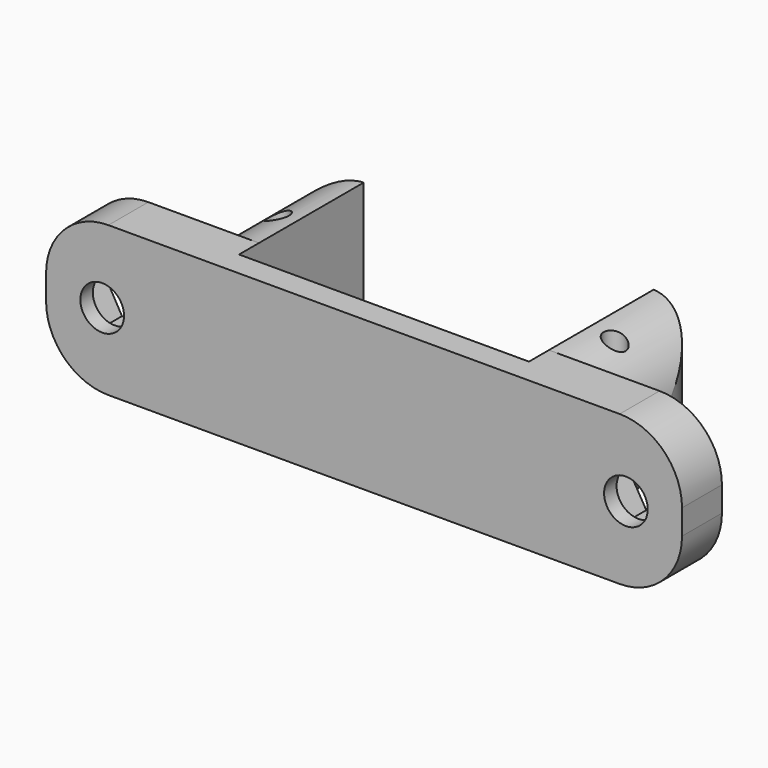
from build123d import *

# Parameters (mm, degrees)
F0_R        = 0.875
F1_DEPTH    = 12
F2_R        = 1.75
F3_DEPTH    = 25
F4_DEPTH    = 6
F5_T1_DEPTH = 36.9921862789
F5_T3_DEPTH = 22.9960931395
F5_T5_DEPTH = 29


# Not quite as in the source:
# - a fillet or chamfer that OpenCascade refuses, or shapes differently, is made with other operations: its cross-section is extruded or revolved along the edge and cut away or added


with BuildPart() as f1:
    # F0 (on Top) → F1 (new body)
    with BuildSketch(Plane.XY):
        Polygon((-11.625, -5.25), (-11.625, 7.25), (-16.5, 7.25), (-16.5, -3.25), (-16.5, -5.25), align=None)
        with Locations((-13.5, 1)):
            Circle(F0_R, mode=Mode.SUBTRACT)
        Polygon((-16.5, -5.25), (-16.5, -3.25), (-25.5, -3.25), (-25.5, -7.25), (-16.5, -7.25), align=None)
        Polygon((16.5, -3.25), (16.5, 7.25), (11.625, 7.25), (11.625, -5.25), (16.5, -5.25), align=None)
        with Locations((13.5, 1)):
            Circle(F0_R, mode=Mode.SUBTRACT)
        Polygon((25.5, -3.25), (16.5, -3.25), (16.5, -5.25), (16.5, -7.25), (25.5, -7.25), align=None)
        Polygon((16.5, -5.25), (11.625, -5.25), (-11.625, -5.25), (-16.5, -5.25), (-16.5, -7.25), (16.5, -7.25), align=None)
    extrude(amount=F1_DEPTH)

    # F2 (on Front) → F3 (cut)
    with BuildSketch(Plane.XZ):
        with Locations((21, 6)):
            Circle(F2_R)
        with Locations((-21, 6)):
            Circle(F2_R)
    extrude(amount=F3_DEPTH, mode=Mode.SUBTRACT)

    # F2 (on Front) → F4 (cut)
    with BuildSketch(Plane.XZ):
        Polygon((17.8246783439, 5.9741985751), (19.4346838614, 3.2371900682), (22.6100055175, 3.2629914931), (24.1753216561, 6.0258014249), (22.5653161386, 8.7628099318), (19.3899944825, 8.7370085069), align=None)
        with Locations((21, 6)):
            Circle(F2_R, mode=Mode.SUBTRACT)
        Polygon((-22.6100055175, 3.2629914931), (-19.4346838614, 3.2371900682), (-17.8246783439, 5.9741985751), (-19.3899944825, 8.7370085069), (-22.5653161386, 8.7628099318), (-24.1753216561, 6.0258014249), align=None)
        with Locations((-21, 6)):
            Circle(F2_R, mode=Mode.SUBTRACT)
    extrude(amount=F4_DEPTH, mode=Mode.SUBTRACT)

    # F5: fillet of radius 5 on 10 edges, made by hand

    # F5_s2 → F5_t1 (cut)
    with BuildSketch(Plane.XY.offset(-12.4960931395)):
        with BuildLine():
            ThreePointArc((-11.625, 7.25), (-15.0794552658, 5.7426227552), (-16.5, 2.2515627442))
            Line((-16.5, 2.2515627442), (-16.5, 7.25))
            Line((-16.5, 7.25), (-11.625, 7.25))
        make_face()
        with BuildLine():
            ThreePointArc((16.5, 2.2515627442), (15.0794552658, 5.7426227552), (11.625, 7.25))
            Line((11.625, 7.25), (16.5, 7.25))
            Line((16.5, 7.25), (16.5, 2.2515627442))
        make_face()
    extrude(amount=F5_T1_DEPTH, mode=Mode.SUBTRACT)

    # F5_s4 → F5_t3 (cut)
    with BuildSketch(Plane.XZ.offset(-19.7460931395)):
        with BuildLine():
            ThreePointArc((11.625, 12), (15.0794552658, 10.4926227552), (16.5, 7.0015627442))
            Line((16.5, 7.0015627442), (16.5, 12))
            Line((16.5, 12), (11.625, 12))
        make_face()
        with BuildLine():
            ThreePointArc((11.625, 0), (15.0794552658, 1.5073772448), (16.5, 4.9984372558))
            Line((16.5, 4.9984372558), (16.5, 0))
            Line((16.5, 0), (11.625, 0))
        make_face()
        with BuildLine():
            ThreePointArc((-11.625, 0), (-15.0794552658, 1.5073772448), (-16.5, 4.9984372558))
            Line((-16.5, 4.9984372558), (-16.5, 0))
            Line((-16.5, 0), (-11.625, 0))
        make_face()
        with BuildLine():
            ThreePointArc((-11.625, 12), (-15.0794552658, 10.4926227552), (-16.5, 7.0015627442))
            Line((-16.5, 7.0015627442), (-16.5, 12))
            Line((-16.5, 12), (-11.625, 12))
        make_face()
    extrude(amount=F5_T3_DEPTH, mode=Mode.SUBTRACT)

    # F5_s6 → F5_t5 (cut)
    with BuildSketch(Plane.XZ.offset(-9.25)):
        with BuildLine():
            ThreePointArc((20.5, 0), (24.0355339059, 1.4644660941), (25.5, 5))
            Line((25.5, 5), (25.5, 0))
            Line((25.5, 0), (20.5, 0))
        make_face()
        with BuildLine():
            ThreePointArc((20.5, 12), (24.0355339059, 10.5355339059), (25.5, 7))
            Line((25.5, 7), (25.5, 12))
            Line((25.5, 12), (20.5, 12))
        make_face()
        with BuildLine():
            ThreePointArc((-20.5, 12), (-24.0355339059, 10.5355339059), (-25.5, 7))
            Line((-25.5, 7), (-25.5, 12))
            Line((-25.5, 12), (-20.5, 12))
        make_face()
        with BuildLine():
            ThreePointArc((-20.5, 0), (-24.0355339059, 1.4644660941), (-25.5, 5))
            Line((-25.5, 5), (-25.5, 0))
            Line((-25.5, 0), (-20.5, 0))
        make_face()
    extrude(amount=F5_T5_DEPTH, mode=Mode.SUBTRACT)


solid = f1.part
